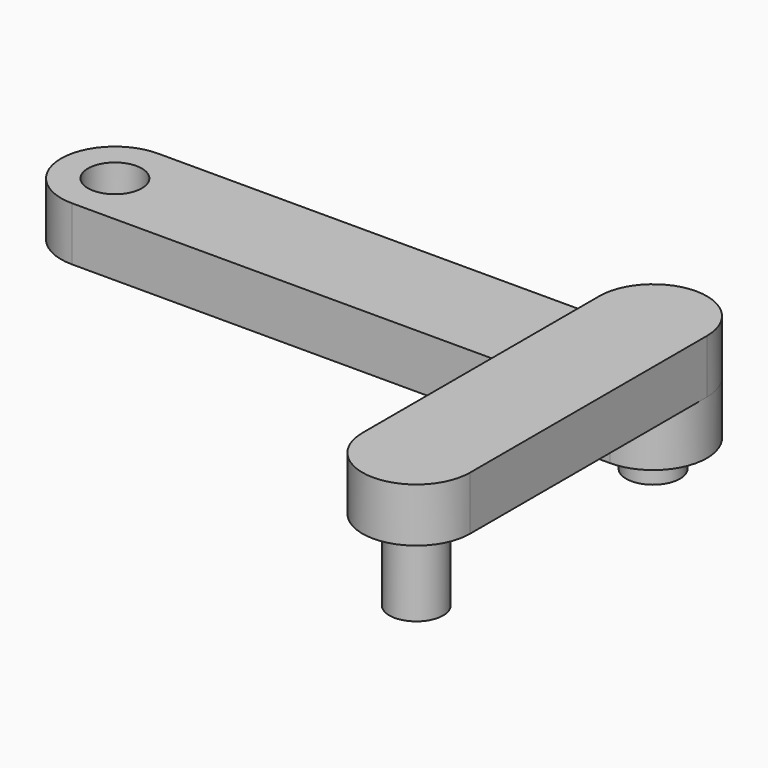
from build123d import *

# Parameters (mm, degrees)
F0_R     = 5
F1_DEPTH = 10
F3_DEPTH = 10
F4_DEPTH = 15
F5_DEPTH = 15


with BuildPart() as f1:
    # F0 (on Top) → F1 (new body)
    with BuildSketch(Plane.XY):
        with BuildLine():
            Line((11.080931966, 0), (-88.919068034, 0))
            ThreePointArc((-88.919068034, 0), (-98.919068034, -10), (-88.919068034, -20))
            Line((-88.919068034, -20), (11.080931966, -20))
            ThreePointArc((11.080931966, -20), (21.080931966, -10), (11.080931966, 0))
        make_face()
        with Locations((-88.919068034, -10)):
            Circle(F0_R, mode=Mode.SUBTRACT)
        with Locations((11.080931966, -10)):
            Circle(F0_R, mode=Mode.SUBTRACT)
    extrude(amount=F1_DEPTH)


with BuildPart() as f3:
    # F2 (on face) → F3 (new body)
    with BuildSketch(Plane.XY.offset(10)):
        with BuildLine():
            Line((21.080931966, -65), (21.080931966, -10))
            ThreePointArc((21.080931966, -10), (18.1519997779, -17.0710678119), (11.080931966, -20))
            Line((11.080931966, -20), (1.080931966, -20))
            Line((1.080931966, -20), (1.080931966, -65))
            ThreePointArc((1.080931966, -65), (11.080931966, -55), (21.080931966, -65))
        make_face()
        with BuildLine():
            ThreePointArc((11.080931966, -20), (18.1519997779, -17.0710678119), (21.080931966, -10))
            Line((21.080931966, -10), (16.080931966, -10))
            ThreePointArc((16.080931966, -10), (11.080931966, -15), (6.080931966, -10))
            Line((6.080931966, -10), (1.080931966, -10))
            ThreePointArc((1.080931966, -10), (4.0098641541, -17.0710678119), (11.080931966, -20))
        make_face()
        with BuildLine():
            Line((1.080931966, -20), (11.080931966, -20))
            ThreePointArc((11.080931966, -20), (4.0098641541, -17.0710678119), (1.080931966, -10))
            Line((1.080931966, -10), (1.080931966, -20))
        make_face()
        with BuildLine():
            Line((16.080931966, -10), (21.080931966, -10))
            ThreePointArc((21.080931966, -10), (18.1519997779, -2.9289321881), (11.080931966, 0))
            ThreePointArc((11.080931966, 0), (4.0098641541, -2.9289321881), (1.080931966, -10))
            Line((1.080931966, -10), (6.080931966, -10))
            ThreePointArc((6.080931966, -10), (11.080931966, -5), (16.080931966, -10))
        make_face()
        with BuildLine():
            ThreePointArc((1.080931966, -65), (11.080931966, -75), (21.080931966, -65))
            ThreePointArc((21.080931966, -65), (11.080931966, -55), (1.080931966, -65))
        make_face()
        with BuildLine():
            ThreePointArc((16.080931966, -65), (11.080931966, -70), (6.080931966, -65))
            ThreePointArc((6.080931966, -65), (11.080931966, -60), (16.080931966, -65))
        make_face(mode=Mode.SUBTRACT)
        with BuildLine():
            ThreePointArc((6.080931966, -10), (11.080931966, -15), (16.080931966, -10))
            Line((16.080931966, -10), (6.080931966, -10))
        make_face()
        with BuildLine():
            Line((6.080931966, -10), (16.080931966, -10))
            ThreePointArc((16.080931966, -10), (11.080931966, -5), (6.080931966, -10))
        make_face()
        with BuildLine():
            ThreePointArc((16.080931966, -65), (11.080931966, -60), (6.080931966, -65))
            Line((6.080931966, -65), (16.080931966, -65))
        make_face()
        with BuildLine():
            Line((16.080931966, -65), (6.080931966, -65))
            ThreePointArc((6.080931966, -65), (11.080931966, -70), (16.080931966, -65))
        make_face()
    extrude(amount=F3_DEPTH)

    # F2 (on face) → F4 (join)
    with BuildSketch(Plane.XY.offset(10)):
        with BuildLine():
            Line((6.080931966, -10), (16.080931966, -10))
            ThreePointArc((16.080931966, -10), (11.080931966, -5), (6.080931966, -10))
        make_face()
        with BuildLine():
            ThreePointArc((6.080931966, -10), (11.080931966, -15), (16.080931966, -10))
            Line((16.080931966, -10), (6.080931966, -10))
        make_face()
    extrude(amount=-F4_DEPTH)

    # F2 (on face) → F5 (join)
    with BuildSketch(Plane.XY.offset(10)):
        with BuildLine():
            Line((16.080931966, -65), (6.080931966, -65))
            ThreePointArc((6.080931966, -65), (11.080931966, -70), (16.080931966, -65))
        make_face()
        with BuildLine():
            ThreePointArc((16.080931966, -65), (11.080931966, -60), (6.080931966, -65))
            Line((6.080931966, -65), (16.080931966, -65))
        make_face()
    extrude(amount=-F5_DEPTH)


solid = Compound([f1.part, f3.part])
